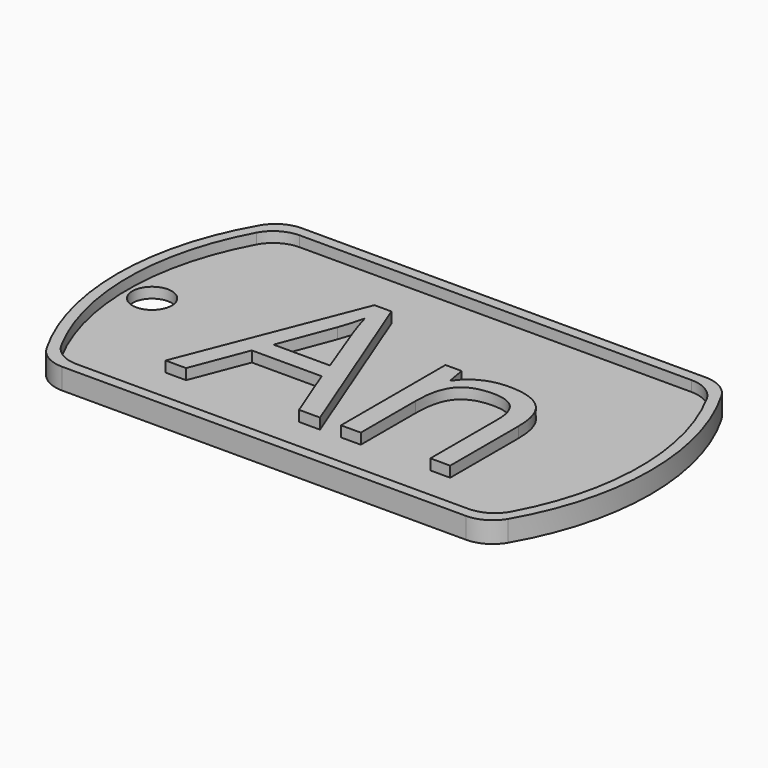
from build123d import *

# Parameters (mm, degrees)
F0_R         = 1.8739594118
F1_DEPTH     = 1
F3_DEPTH     = 1
F4_TEXT_SIZE = 23.2587219216
F5_DEPTH     = 1.016


# Not quite as in the source:
# - Text() gives the source's letters only with a copy of the font that has no kerning and outlines rounded to 1/6400 em; it was checked with that copy


with BuildPart() as f1:
    # F0 (on Top) → F1 (new body)
    with BuildSketch(Plane.XY):
        with BuildLine():
            ThreePointArc((-19.2474145991, 14.2875), (-20.8349145991, 13.862130657), (-21.9970452561, 12.7))
            ThreePointArc((-21.9970452561, 12.7), (-25.4, 0), (-21.9970452561, -12.7))
            ThreePointArc((-21.9970452561, -12.7), (-20.8349145991, -13.862130657), (-19.2474145991, -14.2875))
            Line((-19.2474145991, -14.2875), (19.2474145991, -14.2875))
            ThreePointArc((19.2474145991, -14.2875), (20.8349145991, -13.862130657), (21.9970452561, -12.7))
            ThreePointArc((21.9970452561, -12.7), (25.4, 0), (21.9970452561, 12.7))
            ThreePointArc((21.9970452561, 12.7), (20.8349145991, 13.862130657), (19.2474145991, 14.2875))
            Line((19.2474145991, 14.2875), (-19.2474145991, 14.2875))
        make_face()
        with Locations((-22.0978986472, 0)):
            Circle(F0_R, mode=Mode.SUBTRACT)
    extrude(amount=F1_DEPTH)

    # F2 (on face) → F3 (join)
    with BuildSketch(Plane.XY.offset(1)):
        with BuildLine():
            Line((19.2474145991, 14.2875), (-19.2474145991, 14.2875))
            ThreePointArc((-19.2474145991, 14.2875), (-20.8349145991, 13.862130657), (-21.9970452561, 12.7))
            ThreePointArc((-21.9970452561, 12.7), (-25.4, 0), (-21.9970452561, -12.7))
            ThreePointArc((-21.9970452561, -12.7), (-20.8349145991, -13.862130657), (-19.2474145991, -14.2875))
            Line((-19.2474145991, -14.2875), (19.2474145991, -14.2875))
            ThreePointArc((19.2474145991, -14.2875), (20.8349145991, -13.862130657), (21.9970452561, -12.7))
            ThreePointArc((21.9970452561, -12.7), (25.4, 0), (21.9970452561, 12.7))
            ThreePointArc((21.9970452561, 12.7), (20.8349145991, 13.862130657), (19.2474145991, 14.2875))
        make_face()
        with BuildLine():
            ThreePointArc((-21.4526124879, 11.6252061249), (-20.2856017842, 12.8404540819), (-18.6611352482, 13.2875))
            Line((-18.6611352482, 13.2875), (18.6611352482, 13.2875))
            ThreePointArc((18.6611352482, 13.2875), (20.2856017842, 12.8404540819), (21.4526124879, 11.6252061249))
            ThreePointArc((21.4526124879, 11.6252061249), (24.4, 0), (21.4526124879, -11.6252061249))
            ThreePointArc((21.4526124879, -11.6252061249), (20.2856017842, -12.8404540819), (18.6611352482, -13.2875))
            Line((18.6611352482, -13.2875), (-18.6611352482, -13.2875))
            ThreePointArc((-18.6611352482, -13.2875), (-20.2856017842, -12.8404540819), (-21.4526124879, -11.6252061249))
            ThreePointArc((-21.4526124879, -11.6252061249), (-24.4, 0), (-21.4526124879, 11.6252061249))
        make_face(mode=Mode.SUBTRACT)
    extrude(amount=F3_DEPTH)

    # F4 (on face) → F5 (join)
    with BuildSketch(Plane.XY.offset(1)):
        with Locations((-13.8389393687, -8.7220203131)):
            Text('An', F4_TEXT_SIZE, font='Open Sans', text_align=(TextAlign.LEFT, TextAlign.BOTTOM))
    extrude(amount=F5_DEPTH)


solid = f1.part
